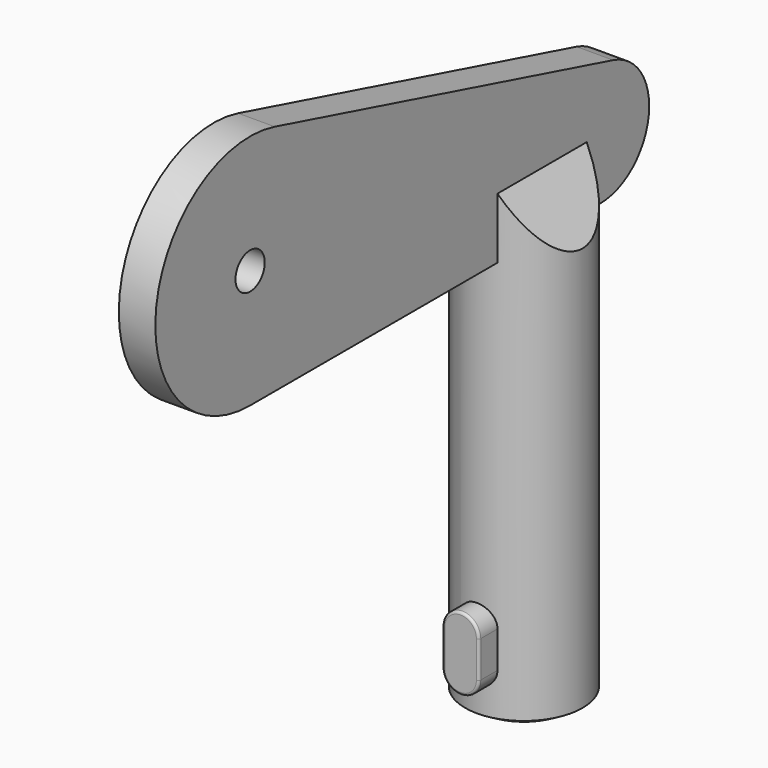
from build123d import *

# Parameters (mm, degrees)
F0_R          = 4.825
F1_DEPTH      = 33
F3_DEPTH      = 6.5
F4_R          = 0.2
F8_DEPTH      = 1.5
F8_DEPTH_BACK = 1.5
F9_T4_DEPTH   = 34.9974315038
F9_S5_R       = 4.825
F9_T6_DEPTH   = 19
F9_T10_DEPTH  = 34.9974315038
F9_S11_R      = 4.825
F9_T12_DEPTH  = 19
F11_R         = 1.5
F12_DEPTH     = 6.3260001


# Not quite as in the source:
# - a fillet or chamfer that OpenCascade refuses, or shapes differently, is made with other operations: its cross-section is extruded or revolved along the edge and cut away or added
# - a feature of the source that left no trace in its solid (it failed there, or was rolled back) is left out


with BuildPart() as f1:
    # F0 (on Top) → F1 (new body)
    with BuildSketch(Plane.XY):
        Circle(F0_R)
    extrude(amount=F1_DEPTH)

    # F2 (on Front) → F3 (join)
    with BuildSketch(Plane.XZ):
        with BuildLine():
            ThreePointArc((-1.5, 3.5), (0, 2), (1.5, 3.5))
            Line((1.5, 3.5), (1.5, 6.5))
            ThreePointArc((1.5, 6.5), (0, 8), (-1.5, 6.5))
            Line((-1.5, 6.5), (-1.5, 3.5))
        make_face()
    extrude(amount=F3_DEPTH)

    # F4
    f4_edges = [f1.edges().sort_by_distance(p)[0] for p in [
        (0, -6.5, 2),
        (1.5, -6.5, 5),
        (0, -6.5, 8),
        (-1.5, -6.5, 5),
    ]]
    fillet(f4_edges, radius=F4_R)

    # F5 (on Front) → F6 (revolve)
    with BuildSketch(Plane.XZ):
        with BuildLine():
            Line((0, 0), (-4.825, 0))
            ThreePointArc((-4.825, 0), (-2.5263919431, -1.1163524169), (0, -1.5))
            Line((0, -1.5), (0, 0))
        make_face()
    revolve(axis=Axis((0, 0, -1.4078605181), (0, 0, -1)))

    # F7 (on Right) → F8 (join, two sides)
    with BuildSketch(Plane.YZ) as f8_sk:
        with BuildLine():
            ThreePointArc((6, 33), (10.9572243069, 37.3473690389), (7.2940952255, 42.8296291314))
            Line((7.2940952255, 42.8296291314), (-27.4792345209, 52.1471147551))
            ThreePointArc((-27.4792345209, 52.1471147551), (-39.6561672268, 44.0107484457), (-30, 33))
            Line((-30, 33), (-6, 33))
            Line((-6, 33), (6, 33))
        make_face()
    extrude(amount=F8_DEPTH)
    extrude(f8_sk.sketch, amount=-F8_DEPTH_BACK)

    # F9: chamfer of 3.5 x 5 on 2 edges, made by hand


with BuildPart() as f9_tool2:
    # F9_s3 → F9_t4 (new body)
    with BuildSketch(Plane.XZ.offset(-17.4987157519)):
        Polygon((5, 33), (1.5, 38), (1.5, 33), align=None)
    extrude(amount=F9_T4_DEPTH)

    # F9_s5 → F9_t6 (intersect, symmetric)
    with BuildSketch(Plane.XY.offset(35.5)):
        Circle(F9_S5_R)
    extrude(amount=F9_T6_DEPTH, both=True, mode=Mode.INTERSECT)


with BuildPart() as f1_1:
    add(f1.part)

    # F9_t1: union F9_tool2
    add(f9_tool2.part)


with BuildPart() as f9_tool8:
    # F9_s9 → F9_t10 (new body)
    with BuildSketch(Plane.XZ.offset(17.4987157519)):
        Polygon((-5, 33), (-1.5, 38), (-1.5, 33), align=None)
    extrude(amount=-F9_T10_DEPTH)

    # F9_s11 → F9_t12 (intersect, symmetric)
    with BuildSketch(Plane.XY.offset(35.5)):
        Circle(F9_S11_R)
    extrude(amount=F9_T12_DEPTH, both=True, mode=Mode.INTERSECT)


with BuildPart() as f1_2:
    add(f1_1.part)

    # F9_t7: union F9_tool8
    add(f9_tool8.part)

    # F11 (on face) → F12 (cut, through all)
    with BuildSketch(Plane.YZ.offset(1.5)):
        with Locations((-30, 42.7394899131)):
            Circle(F11_R)
    extrude(amount=-F12_DEPTH, mode=Mode.SUBTRACT)


solid = f1_2.part
